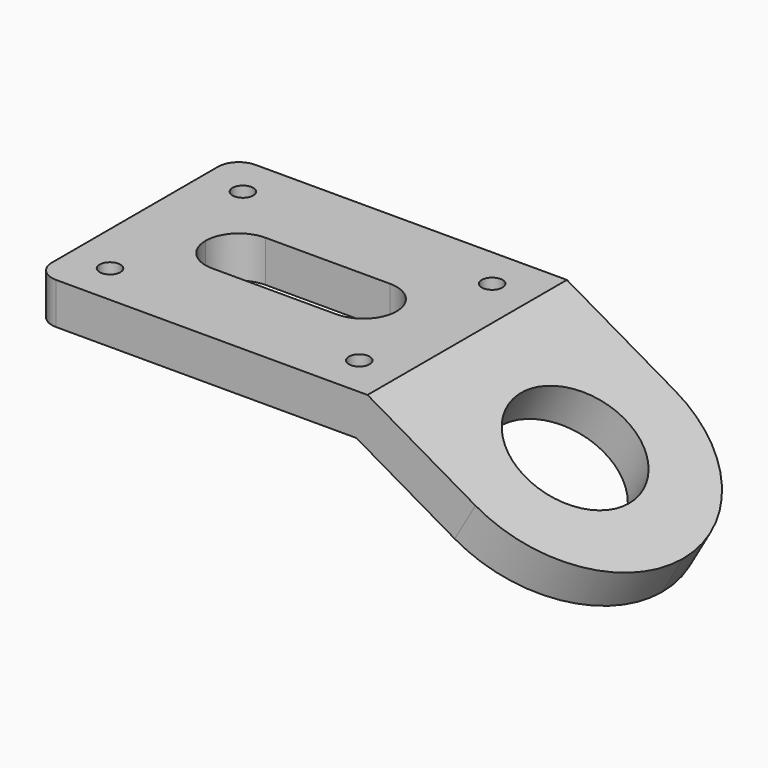
from build123d import *

# Parameters (mm, degrees)
F1_DEPTH = 60
F2_R     = 29.99999
F3_R     = 15
F4_DEPTH = 25
F5_R     = 5
F6_W     = 46
F6_H     = 16
F7_DEPTH = 25
F6_R     = 2.5
F8_DEPTH = 25
F9_R     = 7.99999


# Not quite as in the source:
# - a fillet or chamfer is up to 0.001 mm smaller than in the source, because OpenCascade refuses the exact size


with BuildPart() as f1:
    # F0 (on Front) → F1 (new body)
    with BuildSketch(Plane.XZ):
        Polygon((80, 0), (0, 0), (0, -10), (77.3205080757, -10), align=None)
        Polygon((131.9615242271, -30), (80, 0), (77.3205080757, -10), (126.9615242271, -38.6602540378), align=None)
    extrude(amount=F1_DEPTH)

    # F2 (radius 30 in the source; OpenCascade refuses exactly that, so slightly less here)
    f2_edges = [f1.edges().sort_by_distance(p)[0] for p in [
        (129.461524, 0, -34.330127),
        (129.461524, -60, -34.330127),
    ]]
    fillet(f2_edges, radius=F2_R)

    # F3 (on face) → F4 (cut)
    with BuildSketch(Plane(origin=(20, 0, 34.6410161514), x_dir=(0.8660254038, 0, -0.5), z_dir=(0.5, 0, 0.8660254038))):
        with Locations((99.2820323028, -30)):
            Circle(F3_R)
    extrude(amount=-F4_DEPTH, mode=Mode.SUBTRACT)

    # F5
    f5_edges = [f1.edges().sort_by_distance(p)[0] for p in [
        (0, 0, -5),
        (0, -60, -5),
    ]]
    fillet(f5_edges, radius=F5_R)

    # F6 (on face) → F7 (cut)
    with BuildSketch(Plane.XY):
        with Locations((40, -30)):
            Rectangle(F6_W, F6_H)
    extrude(amount=-F7_DEPTH, mode=Mode.SUBTRACT)

    # F6 (on face) → F8 (cut)
    with BuildSketch(Plane.XY):
        with Locations((10, -50)):
            Circle(F6_R)
        with Locations((70, -50)):
            Circle(F6_R)
        with Locations((70, -10)):
            Circle(F6_R)
        with Locations((10, -10)):
            Circle(F6_R)
        with Locations((40, -30)):
            Rectangle(F6_W, F6_H)
    extrude(amount=-F8_DEPTH, mode=Mode.SUBTRACT)

    # F9 (radius 8 in the source; OpenCascade refuses exactly that, so slightly less here)
    f9_edges = [f1.edges().sort_by_distance(p)[0] for p in [
        (63, -22, -5),
        (63, -38, -5),
        (17, -22, -5),
        (17, -38, -5),
    ]]
    fillet(f9_edges, radius=F9_R)


solid = f1.part
